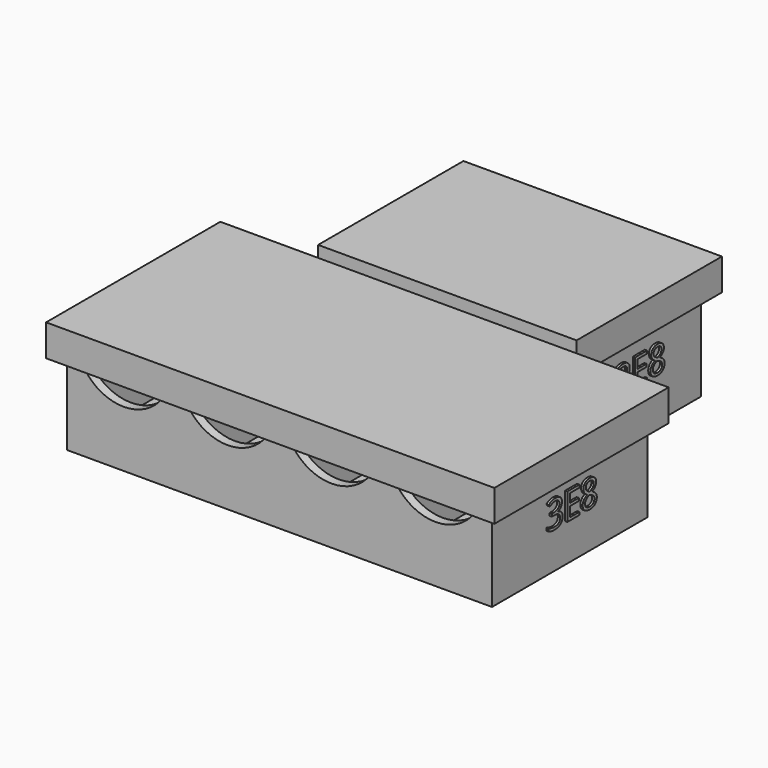
from build123d import *

# Parameters (mm, degrees)
F0_W          = 94
F0_H          = 43
F1_DEPTH      = 2
F0_W_2        = 52
F0_H_2        = 35
F2_W          = 94
F2_H          = 43
F2_W_2        = 21
F2_H_2        = 39
F3_DEPTH      = 21
F5_DEPTH      = 84.001
F7_W          = 99.2
F7_H          = 48.2
F8_DEPTH      = 2
F9_W          = 99.2
F9_H          = 48.2
F9_W_2        = 95.2
F9_H_2        = 44.2
F10_DEPTH     = 5
F11_W         = 52
F11_H         = 35
F11_W_2       = 23
F11_H_2       = 31
F12_DEPTH     = 23
F14_DEPTH     = 35.001
F16_W         = 57.2
F16_H         = 40.2
F17_DEPTH     = 2
F18_W         = 57.2
F18_H         = 40.2
F18_W_2       = 53.2
F18_H_2       = 36.2
F19_DEPTH     = 5
F20_TEXT_SIZE = 8.3333333333
F21_DEPTH     = 0.5
F22_TEXT_SIZE = 8.3333333333
F23_DEPTH     = 0.5


# Not quite as in the source:
# - Text() gives the source's letters only with a copy of the font that has no kerning and outlines rounded to 1/6400 em; it was checked with that copy


with BuildPart() as f1:
    # F0 (on Top) → F1 (new body)
    with BuildSketch(Plane.XY):
        Rectangle(F0_W, F0_H)
    extrude(amount=F1_DEPTH)

    # F2 (on face) → F3 (join)
    with BuildSketch(Plane.XY.offset(2)):
        Rectangle(F2_W, F2_H)
        with Locations((-34.5, 0)):
            Rectangle(F2_W_2, F2_H_2, mode=Mode.SUBTRACT)
        with Locations((-11.5, 0)):
            Rectangle(F2_W_2, F2_H_2, mode=Mode.SUBTRACT)
        with Locations((11.5, 0)):
            Rectangle(F2_W_2, F2_H_2, mode=Mode.SUBTRACT)
        with Locations((34.5, 0)):
            Rectangle(F2_W_2, F2_H_2, mode=Mode.SUBTRACT)
    extrude(amount=F3_DEPTH)

    # F4 (on face) → F5 (cut, through all)
    with BuildSketch(Plane.XZ.offset(21.5)):
        with BuildLine():
            Line((-24, 23), (-45, 23))
            ThreePointArc((-45, 23), (-34.5, 12.5), (-24, 23))
        make_face()
        with BuildLine():
            Line((-1, 23), (-22, 23))
            ThreePointArc((-22, 23), (-11.5, 12.5), (-1, 23))
        make_face()
        with BuildLine():
            Line((22, 23), (1, 23))
            ThreePointArc((1, 23), (11.5, 12.5), (22, 23))
        make_face()
        with BuildLine():
            Line((45, 23), (24, 23))
            ThreePointArc((24, 23), (34.5, 12.5), (45, 23))
        make_face()
    extrude(amount=-F5_DEPTH, mode=Mode.SUBTRACT)

    # F20 (on face) → F21 (join)
    with BuildSketch(Plane.YZ.offset(47)):
        with Locations((-6.8658854167, 8.5)):
            Text('3E8', F20_TEXT_SIZE, font='Open Sans', text_align=(TextAlign.LEFT, TextAlign.BOTTOM))
    extrude(amount=F21_DEPTH)


with BuildPart() as f1b:
    # F0 (on Top) → F1, piece 2 (new body)
    with BuildSketch(Plane.XY):
        with Locations((0, 45)):
            Rectangle(F0_W_2, F0_H_2)
    extrude(amount=F1_DEPTH)

    # F11 (on face) → F12 (join)
    with BuildSketch(Plane.XY.offset(2)):
        with Locations((0, 45)):
            Rectangle(F11_W, F11_H)
        with Locations((-12.5, 45)):
            Rectangle(F11_W_2, F11_H_2, mode=Mode.SUBTRACT)
        with Locations((12.5, 45)):
            Rectangle(F11_W_2, F11_H_2, mode=Mode.SUBTRACT)
    extrude(amount=F12_DEPTH)

    # F13 (on face) → F14 (cut, through all)
    with BuildSketch(Plane.XZ.offset(-27.5)):
        with BuildLine():
            Line((-1, 25), (-24, 25))
            ThreePointArc((-24, 25), (-12.5, 13.5), (-1, 25))
        make_face()
        with BuildLine():
            Line((24, 25), (1, 25))
            ThreePointArc((1, 25), (12.5, 13.5), (24, 25))
        make_face()
    extrude(amount=-F14_DEPTH, mode=Mode.SUBTRACT)

    # F22 (on face) → F23 (join)
    with BuildSketch(Plane.YZ.offset(26)):
        with Locations((38.1341145833, 9.5)):
            Text('3E8', F22_TEXT_SIZE, font='Open Sans', text_align=(TextAlign.LEFT, TextAlign.BOTTOM))
    extrude(amount=F23_DEPTH)


with BuildPart() as f8:
    # F7 (on offset) → F8 (new body)
    with BuildSketch(Plane.XY.offset(23.1)):
        Rectangle(F7_W, F7_H)
    extrude(amount=F8_DEPTH)

    # F9 (on face) → F10 (join)
    with BuildSketch(Plane(origin=(0, 0, 23.1), x_dir=(1, 0, 0), z_dir=(0, 0, -1))):
        Rectangle(F9_W, F9_H)
        Rectangle(F9_W_2, F9_H_2, mode=Mode.SUBTRACT)
    extrude(amount=F10_DEPTH)


with BuildPart() as f17:
    # F16 (on offset) → F17 (new body)
    with BuildSketch(Plane.XY.offset(25.1)):
        with Locations((0, 45)):
            Rectangle(F16_W, F16_H)
    extrude(amount=F17_DEPTH)

    # F18 (on face) → F19 (join)
    with BuildSketch(Plane(origin=(0, 0, 25.1), x_dir=(1, 0, 0), z_dir=(0, 0, -1))):
        with Locations((0, -45)):
            Rectangle(F18_W, F18_H)
        with Locations((0, -45)):
            Rectangle(F18_W_2, F18_H_2, mode=Mode.SUBTRACT)
    extrude(amount=F19_DEPTH)


solid = Compound([f1.part, f1b.part, f8.part, f17.part])
